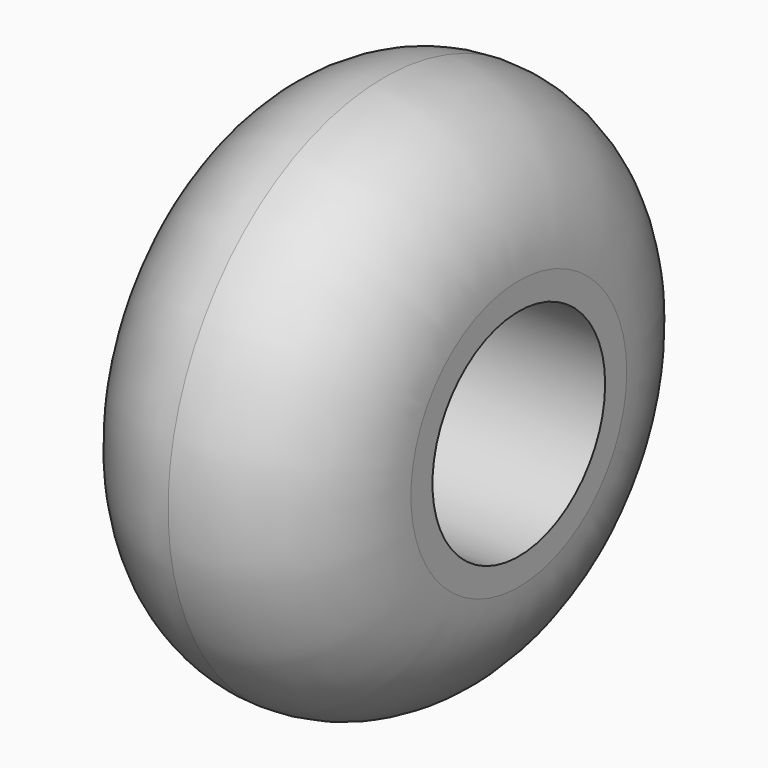
from build123d import *

# Parameters (mm, degrees)
F0_R     = 10
F0_R_2   = 4
F1_DEPTH = 10
F2_R     = 4.99999


# Not quite as in the source:
# - a fillet or chamfer is up to 0.001 mm smaller than in the source, because OpenCascade refuses the exact size


with BuildPart() as f1:
    # F0 (on Right) → F1 (new body)
    with BuildSketch(Plane.YZ):
        Circle(F0_R)
        Circle(F0_R_2, mode=Mode.SUBTRACT)
    extrude(amount=F1_DEPTH)

    # F2 (radius 5 in the source; OpenCascade refuses exactly that, so slightly less here)
    f2_edges = [f1.edges().sort_by_distance(p)[0] for p in [
        (10, -10, 0),
        (0, -10, 0),
    ]]
    fillet(f2_edges, radius=F2_R)


solid = f1.part
